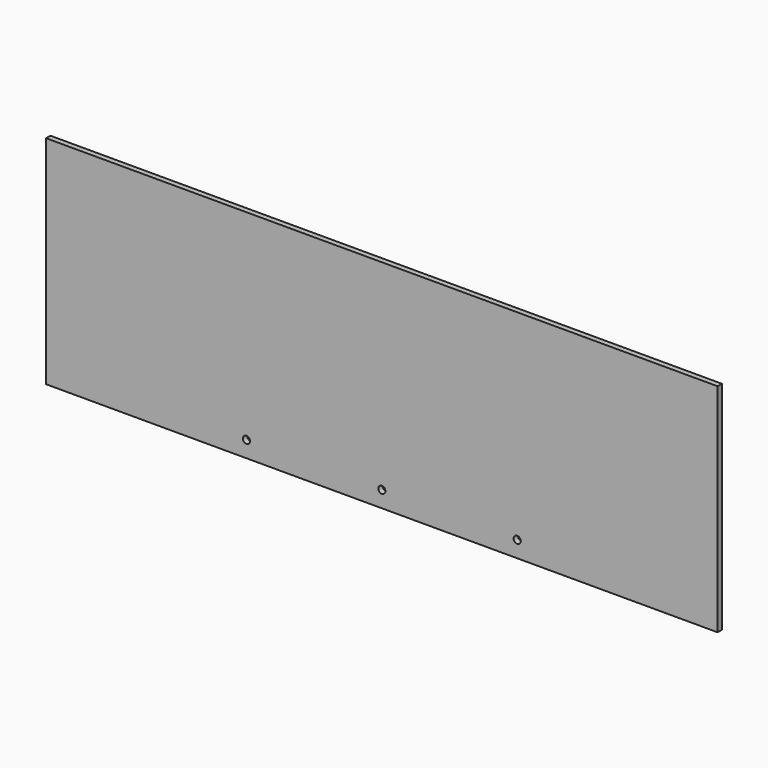
from build123d import *

# Parameters (mm, degrees)
F1_DEPTH = 5
F3_D     = 6.6


# Not quite as in the source:
# - a feature names something its author has since deleted; it is built from what else it names


with BuildPart() as f1:
    # F0 (on Front) → F1 (new body)
    with BuildSketch(Plane.XZ):
        Polygon((-250, 100), (-310, 100), (-310, -100), (310, -100), (310, 100), align=None)
    extrude(amount=F1_DEPTH)

    # F3 (through all)
    with Locations(Plane.XZ.offset(5)):
        with Locations((-125, -85), (125, -85), (0, -85)):
            Hole(F3_D / 2)


solid = f1.part
